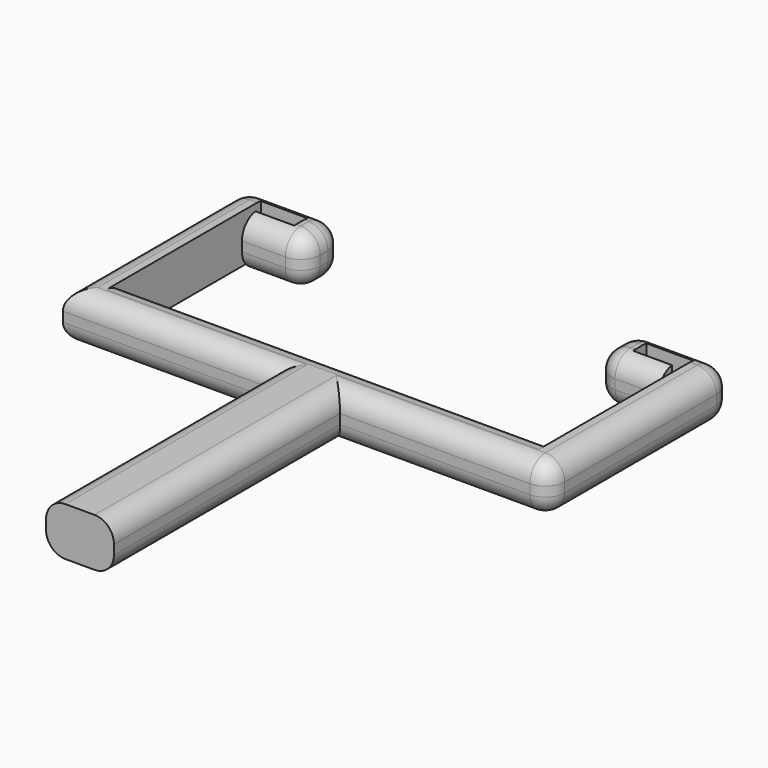
from build123d import *

# Parameters (mm, degrees)
F1_DEPTH      = 6.35
F2_F1_R       = 2.54
F2_F2_R       = 2.54
F2_F3_R       = 2.54
F2_T4_DEPTH   = 16.6182092851
F2_T6_DEPTH   = 1.27
F2_T9_ANGLE   = 90
F2_T11_ANGLE  = 90
F3_T1_DEPTH   = 5.693692497
F3_T3_DEPTH   = 1.2540775669
F3_T5_DEPTH   = 7.7282092851
F3_T7_DEPTH   = 1.27
F3_T9_DEPTH   = 24.9126996231
F3_T11_DEPTH  = 24.9219618431
F3_T13_DEPTH  = 37.0918661356
F3_T15_DEPTH  = 27.4619618431
F3_T17_DEPTH  = 27.4526996231
F3_T19_DEPTH  = 56.7609667778
F3_S23_W      = 2.5908
F3_S23_H      = 2.5908
F3_T24_DEPTH  = 2.5908
F3_S29_W      = 2.5908
F3_S29_H      = 2.5908
F3_T30_DEPTH  = 2.5908
F3_S35_W      = 2.5908
F3_S35_H      = 2.5908
F3_T36_DEPTH  = 2.5908
F3_S41_W      = 2.5908
F3_S41_H      = 2.5908
F3_T42_DEPTH  = 2.5908
F3_S47_W      = 2.5908
F3_S47_H      = 2.5908
F3_T48_DEPTH  = 2.5908
F3_S53_W      = 2.5908
F3_S53_H      = 2.5908
F3_T54_DEPTH  = 2.5908
F3_S59_W      = 2.5908
F3_S59_H      = 2.5908
F3_T60_DEPTH  = 2.5908
F3_S65_W      = 2.5908
F3_S65_H      = 2.5908
F3_T66_DEPTH  = 2.5908
F3_T70_ANGLE  = 90.0000000056
F3_T72_ANGLE  = 90.0000000056
F3_T77_DEPTH  = 31.2719618431
F3_T81_DEPTH  = 43.4418661356
F3_T88_DEPTH  = 43.4418661356
F3_T92_DEPTH  = 33.8119618431
F3_T99_DEPTH  = 33.8119618431
F3_T103_DEPTH = 33.8026996231
F3_T110_DEPTH = 31.2719618431
F3_T114_DEPTH = 43.4418661356
F3_T121_DEPTH = 43.4418661356
F3_T125_DEPTH = 33.8119618431
F3_T132_DEPTH = 33.8119618431
F3_T136_DEPTH = 33.8026996231


# Not quite as in the source:
# - a fillet or chamfer that OpenCascade refuses, or shapes differently, is made with other operations: its cross-section is extruded or revolved along the edge and cut away or added
# - two fillets or chamfers of one size are made in one step


with BuildPart() as f1:
    # F0 (on Top) → F1 (new body)
    with BuildSketch(Plane.XY):
        Polygon((-4.4542392716, -33.3753190935), (0, -33.3753190935), (4.4542392716, -33.3753190935), (4.4542392716, 3.7165470421), (31.9162011147, 3.7165470421), (31.9162011147, 8.9918673038), (31.9162011147, 33.7092466652), (28.3804833889, 33.7092466652), (19.1079918295, 33.7092466652), (19.1079918295, 31.8067148328), (19.1079918295, 27.3751690984), (22.2418643534, 27.3751690984), (27.3416843265, 27.3751690984), (27.3416843265, 29.5909419656), (22.2418643534, 29.5909419656), (22.2418643534, 31.8067148328), (28.3804833889, 31.8067148328), (28.3804833889, 8.9918673038), (4.4542392716, 8.9918673038), (0, 8.9918673038), (-4.4542392716, 8.9918673038), (-28.3804833889, 8.9918673038), (-28.3804833889, 31.8067148328), (-22.2418643534, 31.8067148328), (-22.2418643534, 29.5909419656), (-27.3416843265, 29.5909419656), (-27.3416843265, 27.3751690984), (-22.2418643534, 27.3751690984), (-19.1079918295, 27.3751690984), (-19.1079918295, 31.8067148328), (-19.1079918295, 33.7092466652), (-28.3804833889, 33.7092466652), (-31.9162011147, 33.7092466652), (-31.9162011147, 8.9918673038), (-31.9162011147, 3.7165470421), (-4.4542392716, 3.7165470421), align=None)
    extrude(amount=F1_DEPTH)

    # F2: fillet of radius 2.54 on 7 edges, made by hand

    # F2_f1
    f2_f1_edges = [f1.edges().sort_by_distance(p)[0] for p in [
        (23.224838078, 27.3751690984, 0),
    ]]
    fillet(f2_f1_edges, radius=F2_F1_R)

    # F2_f2
    f2_f2_edges = [f1.edges().sort_by_distance(p)[0] for p in [
        (23.224838078, 27.3751690984, 6.35),
    ]]
    fillet(f2_f2_edges, radius=F2_F2_R)

    # F2_f3
    f2_f3_edges = [f1.edges().sort_by_distance(p)[0] for p in [
        (19.1079918295, 27.3751690984, 3.175),
    ]]
    fillet(f2_f3_edges, radius=F2_F3_R)

    # F2_s5 → F2_t4 (cut)
    with BuildSketch(Plane.YZ.offset(21.6479918295)):
        with BuildLine():
            ThreePointArc((33.7092466652, 2.54), (32.9652978895, 0.7439487758), (31.1692466652, 0))
            Line((31.1692466652, 0), (31.1692466652, -0.0508))
            Line((31.1692466652, -0.0508), (33.7600466652, -0.0508))
            Line((33.7600466652, -0.0508), (33.7600466652, 2.54))
            Line((33.7600466652, 2.54), (33.7092466652, 2.54))
        make_face()
        with BuildLine():
            ThreePointArc((33.7092466652, 3.81), (32.9652978895, 5.6060512242), (31.1692466652, 6.35))
            Line((31.1692466652, 6.35), (31.1692466652, 6.4008))
            Line((31.1692466652, 6.4008), (33.7600466652, 6.4008))
            Line((33.7600466652, 6.4008), (33.7600466652, 3.81))
            Line((33.7600466652, 3.81), (33.7092466652, 3.81))
        make_face()
    extrude(amount=F2_T4_DEPTH, mode=Mode.SUBTRACT)

    # F2_s7 → F2_t6 (cut)
    with BuildSketch(Plane.XY.offset(2.54)):
        with BuildLine():
            ThreePointArc((19.1079918295, 31.1692466652), (19.8519406053, 32.9652978895), (21.6479918295, 33.7092466652))
            Line((21.6479918295, 33.7092466652), (21.6479918295, 33.7600466652))
            Line((21.6479918295, 33.7600466652), (19.0571918295, 33.7600466652))
            Line((19.0571918295, 33.7600466652), (19.0571918295, 31.1692466652))
            Line((19.0571918295, 31.1692466652), (19.1079918295, 31.1692466652))
        make_face()
    extrude(amount=F2_T6_DEPTH, mode=Mode.SUBTRACT)

    # F2_s8 → F2_t9 (revolve, cut)
    with BuildSketch(Plane.XY.offset(2.54)):
        with BuildLine():
            ThreePointArc((21.6479918295, 33.7092466652), (19.8519406053, 32.9652978895), (19.1079918295, 31.1692466652))
            Line((19.1079918295, 31.1692466652), (19.0571918295, 31.1692466652))
            Line((19.0571918295, 31.1692466652), (19.0571918295, 33.7600466652))
            Line((19.0571918295, 33.7600466652), (21.6479918295, 33.7600466652))
            Line((21.6479918295, 33.7600466652), (21.6479918295, 33.7092466652))
        make_face()
    revolve(axis=Axis((21.6479918295, 33.7092466652, 2.54), (0, -1, 0)), revolution_arc=F2_T9_ANGLE, mode=Mode.SUBTRACT)

    # F2_s10 → F2_t11 (revolve, cut)
    with BuildSketch(Plane.XY.offset(3.81)):
        with BuildLine():
            ThreePointArc((21.6479918295, 33.7092466652), (19.8519406053, 32.9652978895), (19.1079918295, 31.1692466652))
            Line((19.1079918295, 31.1692466652), (19.0571918295, 31.1692466652))
            Line((19.0571918295, 31.1692466652), (19.0571918295, 33.7600466652))
            Line((19.0571918295, 33.7600466652), (21.6479918295, 33.7600466652))
            Line((21.6479918295, 33.7600466652), (21.6479918295, 33.7092466652))
        make_face()
    revolve(axis=Axis((21.6479918295, 33.7092466652, 3.81), (0, 1, 0)), revolution_arc=F2_T11_ANGLE, mode=Mode.SUBTRACT)

    # F3: fillet of radius 2.54 on 27 edges, made by hand

    # F3_s2 → F3_t1 (cut)
    with BuildSketch(Plane.YZ.offset(-27.3416843265)):
        with BuildLine():
            ThreePointArc((29.9151690984, 0), (28.1191178742, 0.7439487758), (27.3751690984, 2.54))
            Line((27.3751690984, 2.54), (27.3243690984, 2.54))
            Line((27.3243690984, 2.54), (27.3243690984, -0.0508))
            Line((27.3243690984, -0.0508), (29.9151690984, -0.0508))
            Line((29.9151690984, -0.0508), (29.9151690984, 0))
        make_face()
        with BuildLine():
            ThreePointArc((29.9151690984, 6.35), (28.1191178742, 5.6060512242), (27.3751690984, 3.81))
            Line((27.3751690984, 3.81), (27.3243690984, 3.81))
            Line((27.3243690984, 3.81), (27.3243690984, 6.4008))
            Line((27.3243690984, 6.4008), (29.9151690984, 6.4008))
            Line((29.9151690984, 6.4008), (29.9151690984, 6.35))
        make_face()
    extrude(amount=F3_T1_DEPTH, mode=Mode.SUBTRACT)

    # F3_s4 → F3_t3 (cut)
    with BuildSketch(Plane.XZ.offset(-31.1692466652)):
        with BuildLine():
            ThreePointArc((-21.6479918295, 6.35), (-19.8519406053, 5.6060512242), (-19.1079918295, 3.81))
            Line((-19.1079918295, 3.81), (-19.0571918295, 3.81))
            Line((-19.0571918295, 3.81), (-19.0571918295, 6.4008))
            Line((-19.0571918295, 6.4008), (-21.6479918295, 6.4008))
            Line((-21.6479918295, 6.4008), (-21.6479918295, 6.35))
        make_face()
        with BuildLine():
            ThreePointArc((-21.6479918295, 0), (-19.8519406053, 0.7439487758), (-19.1079918295, 2.54))
            Line((-19.1079918295, 2.54), (-19.0571918295, 2.54))
            Line((-19.0571918295, 2.54), (-19.0571918295, -0.0508))
            Line((-19.0571918295, -0.0508), (-21.6479918295, -0.0508))
            Line((-21.6479918295, -0.0508), (-21.6479918295, 0))
        make_face()
    extrude(amount=F3_T3_DEPTH, mode=Mode.SUBTRACT)

    # F3_s6 → F3_t5 (cut)
    with BuildSketch(Plane.YZ.offset(-29.3762011147)):
        with BuildLine():
            ThreePointArc((31.1692466652, 6.35), (32.9652978895, 5.6060512242), (33.7092466652, 3.81))
            Line((33.7092466652, 3.81), (33.7600466652, 3.81))
            Line((33.7600466652, 3.81), (33.7600466652, 6.4008))
            Line((33.7600466652, 6.4008), (31.1692466652, 6.4008))
            Line((31.1692466652, 6.4008), (31.1692466652, 6.35))
        make_face()
        with BuildLine():
            ThreePointArc((31.1692466652, 0), (32.9652978895, 0.7439487758), (33.7092466652, 2.54))
            Line((33.7092466652, 2.54), (33.7600466652, 2.54))
            Line((33.7600466652, 2.54), (33.7600466652, -0.0508))
            Line((33.7600466652, -0.0508), (31.1692466652, -0.0508))
            Line((31.1692466652, -0.0508), (31.1692466652, 0))
        make_face()
    extrude(amount=F3_T5_DEPTH, mode=Mode.SUBTRACT)

    # F3_s8 → F3_t7 (cut)
    with BuildSketch(Plane.XY.offset(2.54)):
        with BuildLine():
            ThreePointArc((-21.6479918295, 33.7092466652), (-19.8519406053, 32.9652978895), (-19.1079918295, 31.1692466652))
            Line((-19.1079918295, 31.1692466652), (-19.0571918295, 31.1692466652))
            Line((-19.0571918295, 31.1692466652), (-19.0571918295, 33.7600466652))
            Line((-19.0571918295, 33.7600466652), (-21.6479918295, 33.7600466652))
            Line((-21.6479918295, 33.7600466652), (-21.6479918295, 33.7092466652))
        make_face()
        with BuildLine():
            ThreePointArc((-31.9162011147, 31.1692466652), (-31.1722523389, 32.9652978895), (-29.3762011147, 33.7092466652))
            Line((-29.3762011147, 33.7092466652), (-29.3762011147, 33.7600466652))
            Line((-29.3762011147, 33.7600466652), (-31.9670011147, 33.7600466652))
            Line((-31.9670011147, 33.7600466652), (-31.9670011147, 31.1692466652))
            Line((-31.9670011147, 31.1692466652), (-31.9162011147, 31.1692466652))
        make_face()
        with BuildLine():
            ThreePointArc((29.3762011147, 33.7092466652), (31.1722523389, 32.9652978895), (31.9162011147, 31.1692466652))
            Line((31.9162011147, 31.1692466652), (31.9670011147, 31.1692466652))
            Line((31.9670011147, 31.1692466652), (31.9670011147, 33.7600466652))
            Line((31.9670011147, 33.7600466652), (29.3762011147, 33.7600466652))
            Line((29.3762011147, 33.7600466652), (29.3762011147, 33.7092466652))
        make_face()
        with BuildLine():
            ThreePointArc((31.9162011147, 6.2565470421), (31.1722523389, 4.4604958179), (29.3762011147, 3.7165470421))
            Line((29.3762011147, 3.7165470421), (29.3762011147, 3.6657470421))
            Line((29.3762011147, 3.6657470421), (31.9670011147, 3.6657470421))
            Line((31.9670011147, 3.6657470421), (31.9670011147, 6.2565470421))
            Line((31.9670011147, 6.2565470421), (31.9162011147, 6.2565470421))
        make_face()
        with BuildLine():
            ThreePointArc((-19.1079918295, 29.9151690984), (-19.8519406053, 28.1191178742), (-21.6479918295, 27.3751690984))
            Line((-21.6479918295, 27.3751690984), (-21.6479918295, 27.3243690984))
            Line((-21.6479918295, 27.3243690984), (-19.0571918295, 27.3243690984))
            Line((-19.0571918295, 27.3243690984), (-19.0571918295, 29.9151690984))
            Line((-19.0571918295, 29.9151690984), (-19.1079918295, 29.9151690984))
        make_face()
    extrude(amount=F3_T7_DEPTH, mode=Mode.SUBTRACT)

    # F3_s10 → F3_t9 (cut)
    with BuildSketch(Plane.XZ.offset(-31.1692466652)):
        with BuildLine():
            ThreePointArc((29.3762011147, 0), (31.1722523389, 0.7439487758), (31.9162011147, 2.54))
            Line((31.9162011147, 2.54), (31.9670011147, 2.54))
            Line((31.9670011147, 2.54), (31.9670011147, -0.0508))
            Line((31.9670011147, -0.0508), (29.3762011147, -0.0508))
            Line((29.3762011147, -0.0508), (29.3762011147, 0))
        make_face()
        with BuildLine():
            ThreePointArc((31.9162011147, 3.81), (31.1722523389, 5.6060512242), (29.3762011147, 6.35))
            Line((29.3762011147, 6.35), (29.3762011147, 6.4008))
            Line((29.3762011147, 6.4008), (31.9670011147, 6.4008))
            Line((31.9670011147, 6.4008), (31.9670011147, 3.81))
            Line((31.9670011147, 3.81), (31.9162011147, 3.81))
        make_face()
    extrude(amount=F3_T9_DEPTH, mode=Mode.SUBTRACT)

    # F3_s12 → F3_t11 (cut)
    with BuildSketch(Plane.YZ.offset(4.4542392716)):
        with BuildLine():
            ThreePointArc((6.2565470421, 0), (4.4604958179, 0.7439487758), (3.7165470421, 2.54))
            Line((3.7165470421, 2.54), (3.6657470421, 2.54))
            Line((3.6657470421, 2.54), (3.6657470421, -0.0508))
            Line((3.6657470421, -0.0508), (6.2565470421, -0.0508))
            Line((6.2565470421, -0.0508), (6.2565470421, 0))
        make_face()
        with BuildLine():
            ThreePointArc((6.2565470421, 6.35), (4.4604958179, 5.6060512242), (3.7165470421, 3.81))
            Line((3.7165470421, 3.81), (3.6657470421, 3.81))
            Line((3.6657470421, 3.81), (3.6657470421, 6.4008))
            Line((3.6657470421, 6.4008), (6.2565470421, 6.4008))
            Line((6.2565470421, 6.4008), (6.2565470421, 6.35))
        make_face()
    extrude(amount=F3_T11_DEPTH, mode=Mode.SUBTRACT)

    # F3_s14 → F3_t13 (cut)
    with BuildSketch(Plane.XZ.offset(-3.7165470421)):
        with BuildLine():
            ThreePointArc((1.9142392716, 0), (3.7102904958, 0.7439487758), (4.4542392716, 2.54))
            Line((4.4542392716, 2.54), (4.5050392716, 2.54))
            Line((4.5050392716, 2.54), (4.5050392716, -0.0508))
            Line((4.5050392716, -0.0508), (1.9142392716, -0.0508))
            Line((1.9142392716, -0.0508), (1.9142392716, 0))
        make_face()
        with BuildLine():
            ThreePointArc((-1.9142392716, 0), (-3.7102904958, 0.7439487758), (-4.4542392716, 2.54))
            Line((-4.4542392716, 2.54), (-4.5050392716, 2.54))
            Line((-4.5050392716, 2.54), (-4.5050392716, -0.0508))
            Line((-4.5050392716, -0.0508), (-1.9142392716, -0.0508))
            Line((-1.9142392716, -0.0508), (-1.9142392716, 0))
        make_face()
        with BuildLine():
            ThreePointArc((1.9142392716, 6.35), (3.7102904958, 5.6060512242), (4.4542392716, 3.81))
            Line((4.4542392716, 3.81), (4.5050392716, 3.81))
            Line((4.5050392716, 3.81), (4.5050392716, 6.4008))
            Line((4.5050392716, 6.4008), (1.9142392716, 6.4008))
            Line((1.9142392716, 6.4008), (1.9142392716, 6.35))
        make_face()
        with BuildLine():
            ThreePointArc((-1.9142392716, 6.35), (-3.7102904958, 5.6060512242), (-4.4542392716, 3.81))
            Line((-4.4542392716, 3.81), (-4.5050392716, 3.81))
            Line((-4.5050392716, 3.81), (-4.5050392716, 6.4008))
            Line((-4.5050392716, 6.4008), (-1.9142392716, 6.4008))
            Line((-1.9142392716, 6.4008), (-1.9142392716, 6.35))
        make_face()
    extrude(amount=F3_T13_DEPTH, mode=Mode.SUBTRACT)

    # F3_s16 → F3_t15 (cut)
    with BuildSketch(Plane.YZ.offset(-31.9162011147)):
        with BuildLine():
            ThreePointArc((6.2565470421, 0), (4.4604958179, 0.7439487758), (3.7165470421, 2.54))
            Line((3.7165470421, 2.54), (3.6657470421, 2.54))
            Line((3.6657470421, 2.54), (3.6657470421, -0.0508))
            Line((3.6657470421, -0.0508), (6.2565470421, -0.0508))
            Line((6.2565470421, -0.0508), (6.2565470421, 0))
        make_face()
        with BuildLine():
            ThreePointArc((6.2565470421, 6.35), (4.4604958179, 5.6060512242), (3.7165470421, 3.81))
            Line((3.7165470421, 3.81), (3.6657470421, 3.81))
            Line((3.6657470421, 3.81), (3.6657470421, 6.4008))
            Line((3.6657470421, 6.4008), (6.2565470421, 6.4008))
            Line((6.2565470421, 6.4008), (6.2565470421, 6.35))
        make_face()
    extrude(amount=F3_T15_DEPTH, mode=Mode.SUBTRACT)

    # F3_s18 → F3_t17 (cut)
    with BuildSketch(Plane.XZ.offset(-31.1692466652)):
        with BuildLine():
            ThreePointArc((-29.3762011147, 0), (-31.1722523389, 0.7439487758), (-31.9162011147, 2.54))
            Line((-31.9162011147, 2.54), (-31.9670011147, 2.54))
            Line((-31.9670011147, 2.54), (-31.9670011147, -0.0508))
            Line((-31.9670011147, -0.0508), (-29.3762011147, -0.0508))
            Line((-29.3762011147, -0.0508), (-29.3762011147, 0))
        make_face()
        with BuildLine():
            ThreePointArc((-29.3762011147, 6.35), (-31.1722523389, 5.6060512242), (-31.9162011147, 3.81))
            Line((-31.9162011147, 3.81), (-31.9670011147, 3.81))
            Line((-31.9670011147, 3.81), (-31.9670011147, 6.4008))
            Line((-31.9670011147, 6.4008), (-29.3762011147, 6.4008))
            Line((-29.3762011147, 6.4008), (-29.3762011147, 6.35))
        make_face()
    extrude(amount=F3_T17_DEPTH, mode=Mode.SUBTRACT)

    # F3_s20 → F3_t19 (cut)
    with BuildSketch(Plane.YZ.offset(-28.3804833889)):
        with BuildLine():
            ThreePointArc((6.4518673038, 0), (8.2479185281, 0.7439487758), (8.9918673038, 2.54))
            Line((8.9918673038, 2.54), (9.0426673038, 2.54))
            Line((9.0426673038, 2.54), (9.0426673038, -0.0508))
            Line((9.0426673038, -0.0508), (6.4518673038, -0.0508))
            Line((6.4518673038, -0.0508), (6.4518673038, 0))
        make_face()
        with BuildLine():
            ThreePointArc((8.9918673038, 3.81), (8.2479185281, 5.6060512242), (6.4518673038, 6.35))
            Line((6.4518673038, 6.35), (6.4518673038, 6.4008))
            Line((6.4518673038, 6.4008), (9.0426673038, 6.4008))
            Line((9.0426673038, 6.4008), (9.0426673038, 3.81))
            Line((9.0426673038, 3.81), (8.9918673038, 3.81))
        make_face()
    extrude(amount=F3_T19_DEPTH, mode=Mode.SUBTRACT)


with BuildPart() as f3_tool22:
    # F3_s23 → F3_t24 (new body)
    with BuildSketch(Plane.YZ.offset(-21.6479918295)):
        with Locations((28.6197690984, 1.2446)):
            Rectangle(F3_S23_W, F3_S23_H)
    extrude(amount=F3_T24_DEPTH)

    # F3_s25 → F3_t26 (revolve, cut)
    with BuildSketch(Plane(origin=(-21.6479918295, 29.9151690984, 2.54), x_dir=(0, 0.7071067812, 0.7071067812), z_dir=(0, 0.7071067812, -0.7071067812))):
        with BuildLine():
            ThreePointArc((0, -2.54), (2.54, 0), (0, 2.54))
            Line((0, 2.54), (0, -2.54))
        make_face()
    revolve(axis=Axis((-21.6479918295, 29.9151690984, 2.54), (1, 0, 0)), mode=Mode.SUBTRACT)


with BuildPart() as f1_1:
    add(f1.part)

    # F3_t21: cut F3_tool22
    add(f3_tool22.part, mode=Mode.SUBTRACT)


with BuildPart() as f3_tool28:
    # F3_s29 → F3_t30 (new body)
    with BuildSketch(Plane.XY.offset(3.81)):
        with Locations((-20.3525918295, 28.6197690984)):
            Rectangle(F3_S29_W, F3_S29_H)
    extrude(amount=F3_T30_DEPTH)

    # F3_s31 → F3_t32 (revolve, cut)
    with BuildSketch(Plane(origin=(-21.6479918295, 29.9151690984, 3.81), x_dir=(-0.7071067812, 0.7071067812, 0), z_dir=(0.7071067812, 0.7071067812, 0))):
        with BuildLine():
            ThreePointArc((0, -2.54), (2.54, 0), (0, 2.54))
            Line((0, 2.54), (0, -2.54))
        make_face()
    revolve(axis=Axis((-21.6479918295, 29.9151690984, 3.81), (0, 0, 1)), mode=Mode.SUBTRACT)


with BuildPart() as f1_2:
    add(f1_1.part)

    # F3_t27: cut F3_tool28
    add(f3_tool28.part, mode=Mode.SUBTRACT)


with BuildPart() as f3_tool34:
    # F3_s35 → F3_t36 (new body)
    with BuildSketch(Plane.XZ.offset(-31.1692466652)):
        with Locations((-20.3525918295, 5.1054)):
            Rectangle(F3_S35_W, F3_S35_H)
    extrude(amount=-F3_T36_DEPTH)

    # F3_s37 → F3_t38 (revolve, cut)
    with BuildSketch(Plane(origin=(-21.6479918295, 31.1692466652, 3.81), x_dir=(-0.7071067812, 0, -0.7071067812), z_dir=(0.7071067812, 0, -0.7071067812))):
        with BuildLine():
            ThreePointArc((0, -2.54), (2.54, 0), (0, 2.54))
            Line((0, 2.54), (0, -2.54))
        make_face()
    revolve(axis=Axis((-21.6479918295, 31.1692466652, 3.81), (0, 1, 0)), mode=Mode.SUBTRACT)


with BuildPart() as f1_3:
    add(f1_2.part)

    # F3_t33: cut F3_tool34
    add(f3_tool34.part, mode=Mode.SUBTRACT)


with BuildPart() as f3_tool40:
    # F3_s41 → F3_t42 (new body)
    with BuildSketch(Plane.XZ.offset(-31.1692466652)):
        with Locations((-20.3525918295, 1.2446)):
            Rectangle(F3_S41_W, F3_S41_H)
    extrude(amount=-F3_T42_DEPTH)

    # F3_s43 → F3_t44 (revolve, cut)
    with BuildSketch(Plane(origin=(-21.6479918295, 31.1692466652, 2.54), x_dir=(-0.7071067812, 0, 0.7071067812), z_dir=(-0.7071067812, 0, -0.7071067812))):
        with BuildLine():
            ThreePointArc((0, -2.54), (2.54, 0), (0, 2.54))
            Line((0, 2.54), (0, -2.54))
        make_face()
    revolve(axis=Axis((-21.6479918295, 31.1692466652, 2.54), (0, 1, 0)), mode=Mode.SUBTRACT)


with BuildPart() as f1_4:
    add(f1_3.part)

    # F3_t39: cut F3_tool40
    add(f3_tool40.part, mode=Mode.SUBTRACT)


with BuildPart() as f3_tool46:
    # F3_s47 → F3_t48 (new body)
    with BuildSketch(Plane.XZ.offset(-31.1692466652)):
        with Locations((-30.6716011147, 5.1054)):
            Rectangle(F3_S47_W, F3_S47_H)
    extrude(amount=-F3_T48_DEPTH)

    # F3_s49 → F3_t50 (revolve, cut)
    with BuildSketch(Plane(origin=(-29.3762011147, 31.1692466652, 3.81), x_dir=(0.7071067812, 0, -0.7071067812), z_dir=(0.7071067812, 0, 0.7071067812))):
        with BuildLine():
            ThreePointArc((0, -2.54), (2.54, 0), (0, 2.54))
            Line((0, 2.54), (0, -2.54))
        make_face()
    revolve(axis=Axis((-29.3762011147, 31.1692466652, 3.81), (0, 1, 0)), mode=Mode.SUBTRACT)


with BuildPart() as f1_5:
    add(f1_4.part)

    # F3_t45: cut F3_tool46
    add(f3_tool46.part, mode=Mode.SUBTRACT)


with BuildPart() as f3_tool52:
    # F3_s53 → F3_t54 (new body)
    with BuildSketch(Plane.XZ.offset(-31.1692466652)):
        with Locations((-30.6716011147, 1.2446)):
            Rectangle(F3_S53_W, F3_S53_H)
    extrude(amount=-F3_T54_DEPTH)

    # F3_s55 → F3_t56 (revolve, cut)
    with BuildSketch(Plane(origin=(-29.3762011147, 31.1692466652, 2.54), x_dir=(0.7071067812, 0, 0.7071067812), z_dir=(-0.7071067812, 0, 0.7071067812))):
        with BuildLine():
            ThreePointArc((0, -2.54), (2.54, 0), (0, 2.54))
            Line((0, 2.54), (0, -2.54))
        make_face()
    revolve(axis=Axis((-29.3762011147, 31.1692466652, 2.54), (0, 1, 0)), mode=Mode.SUBTRACT)


with BuildPart() as f1_6:
    add(f1_5.part)

    # F3_t51: cut F3_tool52
    add(f3_tool52.part, mode=Mode.SUBTRACT)


with BuildPart() as f3_tool58:
    # F3_s59 → F3_t60 (new body)
    with BuildSketch(Plane.XZ.offset(-6.2565470421)):
        with Locations((30.6716011147, 1.2446)):
            Rectangle(F3_S59_W, F3_S59_H)
    extrude(amount=F3_T60_DEPTH)

    # F3_s61 → F3_t62 (revolve, cut)
    with BuildSketch(Plane(origin=(29.3762011147, 6.2565470421, 2.54), x_dir=(-0.7071067812, 0, 0.7071067812), z_dir=(0.7071067812, 0, 0.7071067812))):
        with BuildLine():
            ThreePointArc((0, -2.54), (2.54, 0), (0, 2.54))
            Line((0, 2.54), (0, -2.54))
        make_face()
    revolve(axis=Axis((29.3762011147, 6.2565470421, 2.54), (0, -1, 0)), mode=Mode.SUBTRACT)


with BuildPart() as f1_7:
    add(f1_6.part)

    # F3_t57: cut F3_tool58
    add(f3_tool58.part, mode=Mode.SUBTRACT)


with BuildPart() as f3_tool64:
    # F3_s65 → F3_t66 (new body)
    with BuildSketch(Plane.XY.offset(3.81)):
        with Locations((30.6716011147, 4.9611470421)):
            Rectangle(F3_S65_W, F3_S65_H)
    extrude(amount=F3_T66_DEPTH)

    # F3_s67 → F3_t68 (revolve, cut)
    with BuildSketch(Plane(origin=(29.3762011147, 6.2565470421, 3.81), x_dir=(-0.7071067812, 0.7071067812, 0), z_dir=(0.7071067812, 0.7071067812, 0))):
        with BuildLine():
            ThreePointArc((0, -2.54), (2.54, 0), (0, 2.54))
            Line((0, 2.54), (0, -2.54))
        make_face()
    revolve(axis=Axis((29.3762011147, 6.2565470421, 3.81), (0, 0, 1)), mode=Mode.SUBTRACT)


with BuildPart() as f1_8:
    add(f1_7.part)

    # F3_t63: cut F3_tool64
    add(f3_tool64.part, mode=Mode.SUBTRACT)

    # F3_s69 → F3_t70 (revolve, cut)
    with BuildSketch(Plane.XY.offset(2.5399999999)):
        with BuildLine():
            ThreePointArc((29.3762011147, 33.7092466652), (31.1722523389, 32.9652978894), (31.9162011147, 31.1692466652))
            Line((31.9162011147, 31.1692466652), (31.9670011147, 31.1692466652))
            Line((31.9670011147, 31.1692466652), (31.9670011147, 33.7600466652))
            Line((31.9670011147, 33.7600466652), (29.3762011147, 33.7600466652))
            Line((29.3762011147, 33.7600466652), (29.3762011147, 33.7092466652))
        make_face()
    revolve(axis=Axis((31.9162011147, 31.1692466653, 2.5399999999), (-1, 0, 0)), revolution_arc=F3_T70_ANGLE, mode=Mode.SUBTRACT)

    # F3_s71 → F3_t72 (revolve, cut)
    with BuildSketch(Plane.XZ.offset(-31.1692466653)):
        with BuildLine():
            ThreePointArc((31.9162011147, 3.81), (31.1722523389, 5.6060512242), (29.3762011147, 6.35))
            Line((29.3762011147, 6.35), (29.3762011147, 6.4008))
            Line((29.3762011147, 6.4008), (31.9670011147, 6.4008))
            Line((31.9670011147, 6.4008), (31.9670011147, 3.81))
            Line((31.9670011147, 3.81), (31.9162011147, 3.81))
        make_face()
    revolve(axis=Axis((31.9162011147, 31.1692466653, 3.8100000001), (-1, 0, 0)), revolution_arc=F3_T72_ANGLE, mode=Mode.SUBTRACT)


with BuildPart() as f3_tool75:
    # F3_s76 → F3_t77 (new body)
    with BuildSketch(Plane.YZ.offset(-1.8957607284)):
        with BuildLine():
            ThreePointArc((6.2565470421, 0), (4.4604958179, 0.7439487758), (3.7165470421, 2.54))
            Line((3.7165470421, 2.54), (3.6657470421, 2.54))
            Line((3.6657470421, 2.54), (3.6657470421, -0.0508))
            Line((3.6657470421, -0.0508), (6.2565470421, -0.0508))
            Line((6.2565470421, -0.0508), (6.2565470421, 0))
        make_face()
    extrude(amount=F3_T77_DEPTH)

    split(bisect_by=Plane.YZ.offset(4.4542392716), keep=Keep.BOTTOM)


with BuildPart() as f3_tool79:
    # F3_s80 → F3_t81 (new body)
    with BuildSketch(Plane.XZ.offset(33.3753190935)):
        with BuildLine():
            ThreePointArc((1.9142392716, 0), (3.7102904958, 0.7439487758), (4.4542392716, 2.54))
            Line((4.4542392716, 2.54), (4.5050392716, 2.54))
            Line((4.5050392716, 2.54), (4.5050392716, -0.0508))
            Line((4.5050392716, -0.0508), (1.9142392716, -0.0508))
            Line((1.9142392716, -0.0508), (1.9142392716, 0))
        make_face()
    extrude(amount=-F3_T81_DEPTH)

    split(bisect_by=Plane.XZ.offset(-3.7165470421), keep=Keep.BOTTOM)


with BuildPart() as f3_tool75_1:
    add(f3_tool75.part)

    # F3_t83: intersect F3_tool79
    add(f3_tool79.part, mode=Mode.INTERSECT)


with BuildPart() as f1_9:
    add(f1_8.part)

    # F3_t73: cut F3_tool75
    add(f3_tool75_1.part, mode=Mode.SUBTRACT)


with BuildPart() as f3_tool86:
    # F3_s87 → F3_t88 (new body)
    with BuildSketch(Plane.XZ.offset(-10.0665470421)):
        with BuildLine():
            ThreePointArc((-1.9142392716, 0), (-3.7102904958, 0.7439487758), (-4.4542392716, 2.54))
            Line((-4.4542392716, 2.54), (-4.5050392716, 2.54))
            Line((-4.5050392716, 2.54), (-4.5050392716, -0.0508))
            Line((-4.5050392716, -0.0508), (-1.9142392716, -0.0508))
            Line((-1.9142392716, -0.0508), (-1.9142392716, 0))
        make_face()
    extrude(amount=F3_T88_DEPTH)

    split(bisect_by=Plane.XZ.offset(-3.7165470421), keep=Keep.BOTTOM)


with BuildPart() as f3_tool90:
    # F3_s91 → F3_t92 (new body)
    with BuildSketch(Plane.YZ.offset(-31.9162011147)):
        with BuildLine():
            ThreePointArc((6.2565470421, 0), (4.4604958179, 0.7439487758), (3.7165470421, 2.54))
            Line((3.7165470421, 2.54), (3.6657470421, 2.54))
            Line((3.6657470421, 2.54), (3.6657470421, -0.0508))
            Line((3.6657470421, -0.0508), (6.2565470421, -0.0508))
            Line((6.2565470421, -0.0508), (6.2565470421, 0))
        make_face()
    extrude(amount=F3_T92_DEPTH)

    split(bisect_by=Plane.YZ.offset(-4.4542392716), keep=Keep.TOP)


with BuildPart() as f3_tool86_1:
    add(f3_tool86.part)

    # F3_t94: intersect F3_tool90
    add(f3_tool90.part, mode=Mode.INTERSECT)


with BuildPart() as f1_10:
    add(f1_9.part)

    # F3_t84: cut F3_tool86
    add(f3_tool86_1.part, mode=Mode.SUBTRACT)


with BuildPart() as f3_tool97:
    # F3_s98 → F3_t99 (new body)
    with BuildSketch(Plane.YZ.offset(-38.2662011147)):
        with BuildLine():
            ThreePointArc((6.2565470421, 0), (4.4604958179, 0.7439487758), (3.7165470421, 2.54))
            Line((3.7165470421, 2.54), (3.6657470421, 2.54))
            Line((3.6657470421, 2.54), (3.6657470421, -0.0508))
            Line((3.6657470421, -0.0508), (6.2565470421, -0.0508))
            Line((6.2565470421, -0.0508), (6.2565470421, 0))
        make_face()
    extrude(amount=F3_T99_DEPTH)

    split(bisect_by=Plane.YZ.offset(-31.9162011147), keep=Keep.BOTTOM)


with BuildPart() as f3_tool101:
    # F3_s102 → F3_t103 (new body)
    with BuildSketch(Plane.XZ.offset(-31.1692466652)):
        with BuildLine():
            ThreePointArc((-29.3762011147, 0), (-31.1722523389, 0.7439487758), (-31.9162011147, 2.54))
            Line((-31.9162011147, 2.54), (-31.9670011147, 2.54))
            Line((-31.9670011147, 2.54), (-31.9670011147, -0.0508))
            Line((-31.9670011147, -0.0508), (-29.3762011147, -0.0508))
            Line((-29.3762011147, -0.0508), (-29.3762011147, 0))
        make_face()
    extrude(amount=F3_T103_DEPTH)

    split(bisect_by=Plane.XZ.offset(-3.7165470421), keep=Keep.TOP)


with BuildPart() as f3_tool97_1:
    add(f3_tool97.part)

    # F3_t105: intersect F3_tool101
    add(f3_tool101.part, mode=Mode.INTERSECT)


with BuildPart() as f1_11:
    add(f1_10.part)

    # F3_t95: cut F3_tool97
    add(f3_tool97_1.part, mode=Mode.SUBTRACT)


with BuildPart() as f3_tool108:
    # F3_s109 → F3_t110 (new body)
    with BuildSketch(Plane.YZ.offset(-1.8957607284)):
        with BuildLine():
            ThreePointArc((6.2565470421, 6.35), (4.4604958179, 5.6060512242), (3.7165470421, 3.81))
            Line((3.7165470421, 3.81), (3.6657470421, 3.81))
            Line((3.6657470421, 3.81), (3.6657470421, 6.4008))
            Line((3.6657470421, 6.4008), (6.2565470421, 6.4008))
            Line((6.2565470421, 6.4008), (6.2565470421, 6.35))
        make_face()
    extrude(amount=F3_T110_DEPTH)

    split(bisect_by=Plane.YZ.offset(4.4542392716), keep=Keep.BOTTOM)


with BuildPart() as f3_tool112:
    # F3_s113 → F3_t114 (new body)
    with BuildSketch(Plane.XZ.offset(33.3753190935)):
        with BuildLine():
            ThreePointArc((1.9142392716, 6.35), (3.7102904958, 5.6060512242), (4.4542392716, 3.81))
            Line((4.4542392716, 3.81), (4.5050392716, 3.81))
            Line((4.5050392716, 3.81), (4.5050392716, 6.4008))
            Line((4.5050392716, 6.4008), (1.9142392716, 6.4008))
            Line((1.9142392716, 6.4008), (1.9142392716, 6.35))
        make_face()
    extrude(amount=-F3_T114_DEPTH)

    split(bisect_by=Plane.XZ.offset(-3.7165470421), keep=Keep.BOTTOM)


with BuildPart() as f3_tool108_1:
    add(f3_tool108.part)

    # F3_t116: intersect F3_tool112
    add(f3_tool112.part, mode=Mode.INTERSECT)


with BuildPart() as f1_12:
    add(f1_11.part)

    # F3_t106: cut F3_tool108
    add(f3_tool108_1.part, mode=Mode.SUBTRACT)


with BuildPart() as f3_tool119:
    # F3_s120 → F3_t121 (new body)
    with BuildSketch(Plane.XZ.offset(-10.0665470421)):
        with BuildLine():
            ThreePointArc((-1.9142392716, 6.35), (-3.7102904958, 5.6060512242), (-4.4542392716, 3.81))
            Line((-4.4542392716, 3.81), (-4.5050392716, 3.81))
            Line((-4.5050392716, 3.81), (-4.5050392716, 6.4008))
            Line((-4.5050392716, 6.4008), (-1.9142392716, 6.4008))
            Line((-1.9142392716, 6.4008), (-1.9142392716, 6.35))
        make_face()
    extrude(amount=F3_T121_DEPTH)

    split(bisect_by=Plane.XZ.offset(-3.7165470421), keep=Keep.BOTTOM)


with BuildPart() as f3_tool123:
    # F3_s124 → F3_t125 (new body)
    with BuildSketch(Plane.YZ.offset(-31.9162011147)):
        with BuildLine():
            ThreePointArc((6.2565470421, 6.35), (4.4604958179, 5.6060512242), (3.7165470421, 3.81))
            Line((3.7165470421, 3.81), (3.6657470421, 3.81))
            Line((3.6657470421, 3.81), (3.6657470421, 6.4008))
            Line((3.6657470421, 6.4008), (6.2565470421, 6.4008))
            Line((6.2565470421, 6.4008), (6.2565470421, 6.35))
        make_face()
    extrude(amount=F3_T125_DEPTH)

    split(bisect_by=Plane.YZ.offset(-4.4542392716), keep=Keep.TOP)


with BuildPart() as f3_tool119_1:
    add(f3_tool119.part)

    # F3_t127: intersect F3_tool123
    add(f3_tool123.part, mode=Mode.INTERSECT)


with BuildPart() as f1_13:
    add(f1_12.part)

    # F3_t117: cut F3_tool119
    add(f3_tool119_1.part, mode=Mode.SUBTRACT)


with BuildPart() as f3_tool130:
    # F3_s131 → F3_t132 (new body)
    with BuildSketch(Plane.YZ.offset(-38.2662011147)):
        with BuildLine():
            ThreePointArc((6.2565470421, 6.35), (4.4604958179, 5.6060512242), (3.7165470421, 3.81))
            Line((3.7165470421, 3.81), (3.6657470421, 3.81))
            Line((3.6657470421, 3.81), (3.6657470421, 6.4008))
            Line((3.6657470421, 6.4008), (6.2565470421, 6.4008))
            Line((6.2565470421, 6.4008), (6.2565470421, 6.35))
        make_face()
    extrude(amount=F3_T132_DEPTH)

    split(bisect_by=Plane.YZ.offset(-31.9162011147), keep=Keep.BOTTOM)


with BuildPart() as f3_tool134:
    # F3_s135 → F3_t136 (new body)
    with BuildSketch(Plane.XZ.offset(2.6334529579)):
        with BuildLine():
            ThreePointArc((-29.3762011147, 6.35), (-31.1722523389, 5.6060512242), (-31.9162011147, 3.81))
            Line((-31.9162011147, 3.81), (-31.9670011147, 3.81))
            Line((-31.9670011147, 3.81), (-31.9670011147, 6.4008))
            Line((-31.9670011147, 6.4008), (-29.3762011147, 6.4008))
            Line((-29.3762011147, 6.4008), (-29.3762011147, 6.35))
        make_face()
    extrude(amount=-F3_T136_DEPTH)

    split(bisect_by=Plane.XZ.offset(-3.7165470421), keep=Keep.TOP)


with BuildPart() as f3_tool130_1:
    add(f3_tool130.part)

    # F3_t138: intersect F3_tool134
    add(f3_tool134.part, mode=Mode.INTERSECT)


with BuildPart() as f1_14:
    add(f1_13.part)

    # F3_t128: cut F3_tool130
    add(f3_tool130_1.part, mode=Mode.SUBTRACT)


solid = f1_14.part
